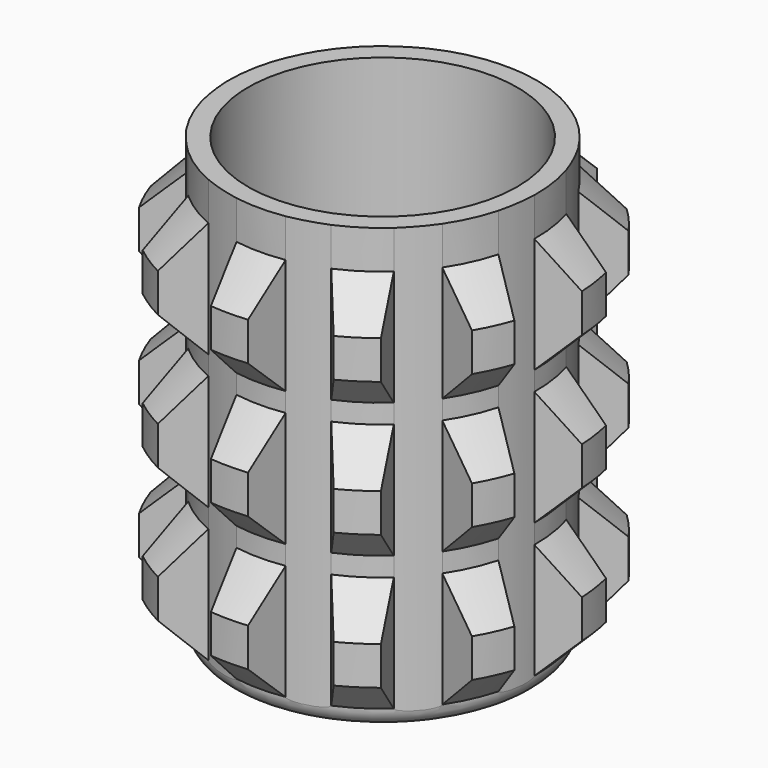
from build123d import *

# Parameters (mm, degrees)
F6_DEPTH = 197.501


# Not quite as in the source:
# - a feature names something its author has since deleted; it is built from what else it names


with BuildPart() as f1:
    # F0 (on Front) → F1 (revolve)
    with BuildSketch(Plane.XZ):
        with BuildLine():
            Line((40, -52.5), (40, 57.5))
            Line((40, 57.5), (35, 57.5))
            Line((35, 57.5), (35, -47.5))
            ThreePointArc((35, -47.5), (33.5355339059, -51.0355339059), (30, -52.5))
            Line((30, -52.5), (0, -52.5))
            Line((0, -52.5), (0, -57.5))
            Line((0, -57.5), (35, -57.5))
            ThreePointArc((35, -57.5), (38.5355339059, -56.0355339059), (40, -52.5))
        make_face()
    revolve(axis=Axis((0, 0, 2.5), (0, 0, 1)))

    # F2 (on Front) → F3 (revolve)
    with BuildSketch(Plane.XZ):
        Polygon((50, 37.5), (40, 47.5), (40, 17.5), (50, 27.5), align=None)
        Polygon((50, -7.5), (50, 2.5), (40, 12.5), (40, -17.5), align=None)
        Polygon((50, -42.5), (50, -32.5), (40, -22.5), (40, -52.5), align=None)
    revolve(axis=Axis((0, 0, 2.5), (0, 0, 1)))

    # F5 (on offset) → F6 (cut, through all)
    with BuildSketch(Plane.XY.offset(140)):
        with BuildLine():
            ThreePointArc((-18.8668219017, 48.0068175713), (-27.9042191508, 43.4198125328), (-35.8309761925, 37.104617598))
            Line((-35.8309761925, 37.104617598), (-25.6622849381, 30.6830104741))
            ThreePointArc((-25.6622849381, 30.6830104741), (-21.591517079, 33.5970563735), (-17.2497496098, 36.0894186487))
            Line((-17.2497496098, 36.0894186487), (-18.8668219017, 48.0068175713))
        make_face()
        with BuildLine():
            ThreePointArc((-5, 39.686269666), (0, 39.9368978106), (5, 39.686269666))
            Line((5, 39.686269666), (10.0826645171, 50.5860788976))
            ThreePointArc((10.0826645171, 50.5860788976), (0, 51.6132305402), (-10.0826645171, 50.5860788976))
            Line((-10.0826645171, 50.5860788976), (-5, 39.686269666))
        make_face()
        with BuildLine():
            ThreePointArc((-41.8262256733, 30.1857308662), (-46.949045883, 21.4409108359), (-50.2032060963, 11.8427023797))
            Line((-50.2032060963, 11.8427023797), (-38.1769757294, 11.9381122525))
            ThreePointArc((-38.1769757294, 11.9381122525), (-36.3278800438, 16.5903869233), (-34.0228255994, 21.0344322061))
            Line((-34.0228255994, 21.0344322061), (-41.8262256733, 30.1857308662))
        make_face()
        with BuildLine():
            ThreePointArc((-51.5060983236, 2.7808878932), (-51.0878822734, -7.3453285571), (-48.6362727834, -17.1791871675))
            Line((-48.6362727834, -17.1791871675), (-38.5707464723, -10.5970522586))
            ThreePointArc((-38.5707464723, -10.5970522586), (-39.5303977752, -5.6836131531), (-39.993894855, -0.6988378398))
            Line((-39.993894855, -0.6988378398), (-51.5060983236, 2.7808878932))
        make_face()
        with BuildLine():
            ThreePointArc((-44.8331486809, -25.5068673371), (-39.0066770118, -33.7994780328), (-31.6276665093, -40.7468061715))
            Line((-31.6276665093, -40.7468061715), (-26.718577738, -29.7677275528))
            ThreePointArc((-26.718577738, -29.7677275528), (-30.1822935214, -26.1531062118), (-33.2671850775, -22.2102318092))
            Line((-33.2671850775, -22.2102318092), (-44.8331486809, -25.5068673371))
        make_face()
        with BuildLine():
            ThreePointArc((-23.9259911079, -45.6963724108), (-14.5411274069, -49.5225320489), (-4.5774995889, -51.3776021191))
            Line((-4.5774995889, -51.3776021191), (-6.3834493564, -39.4873596777))
            ThreePointArc((-6.3834493564, -39.4873596777), (-11.2515243325, -38.3191728373), (-15.9783790926, -36.6700341093))
            Line((-15.9783790926, -36.6700341093), (-23.9259911079, -45.6963724108))
        make_face()
        with BuildLine():
            ThreePointArc((4.5774995889, -51.3776021191), (14.5411274069, -49.5225320489), (23.9259911079, -45.6963724108))
            Line((23.9259911079, -45.6963724108), (15.9783790926, -36.6700341093))
            ThreePointArc((15.9783790926, -36.6700341093), (11.2515243325, -38.3191728373), (6.3834493564, -39.4873596777))
            Line((6.3834493564, -39.4873596777), (4.5774995889, -51.3776021191))
        make_face()
        with BuildLine():
            ThreePointArc((31.6276665093, -40.7468061715), (39.0066770118, -33.7994780328), (44.8331486809, -25.5068673371))
            Line((44.8331486809, -25.5068673371), (33.2671850775, -22.2102318092))
            ThreePointArc((33.2671850775, -22.2102318092), (30.1822935214, -26.1531062118), (26.718577738, -29.7677275528))
            Line((26.718577738, -29.7677275528), (31.6276665093, -40.7468061715))
        make_face()
        with BuildLine():
            ThreePointArc((48.6362727834, -17.1791871675), (51.0878822734, -7.3453285571), (51.5060983236, 2.7808878932))
            Line((51.5060983236, 2.7808878932), (39.993894855, -0.6988378398))
            ThreePointArc((39.993894855, -0.6988378398), (39.5303977752, -5.6836131531), (38.5707464723, -10.5970522586))
            Line((38.5707464723, -10.5970522586), (48.6362727834, -17.1791871675))
        make_face()
        with BuildLine():
            ThreePointArc((50.2032060963, 11.8427023797), (46.949045883, 21.4409108359), (41.8262256733, 30.1857308662))
            Line((41.8262256733, 30.1857308662), (34.0228255994, 21.0344322061))
            ThreePointArc((34.0228255994, 21.0344322061), (36.3278800438, 16.5903869233), (38.1769757294, 11.9381122525))
            Line((38.1769757294, 11.9381122525), (50.2032060963, 11.8427023797))
        make_face()
        with BuildLine():
            ThreePointArc((35.8309761925, 37.104617598), (27.9042191508, 43.4198125328), (18.8668219017, 48.0068175713))
            Line((18.8668219017, 48.0068175713), (17.2497496098, 36.0894186487))
            ThreePointArc((17.2497496098, 36.0894186487), (21.591517079, 33.5970563735), (25.6622849381, 30.6830104741))
            Line((25.6622849381, 30.6830104741), (35.8309761925, 37.104617598))
        make_face()
    extrude(amount=-F6_DEPTH, mode=Mode.SUBTRACT)


solid = f1.part
